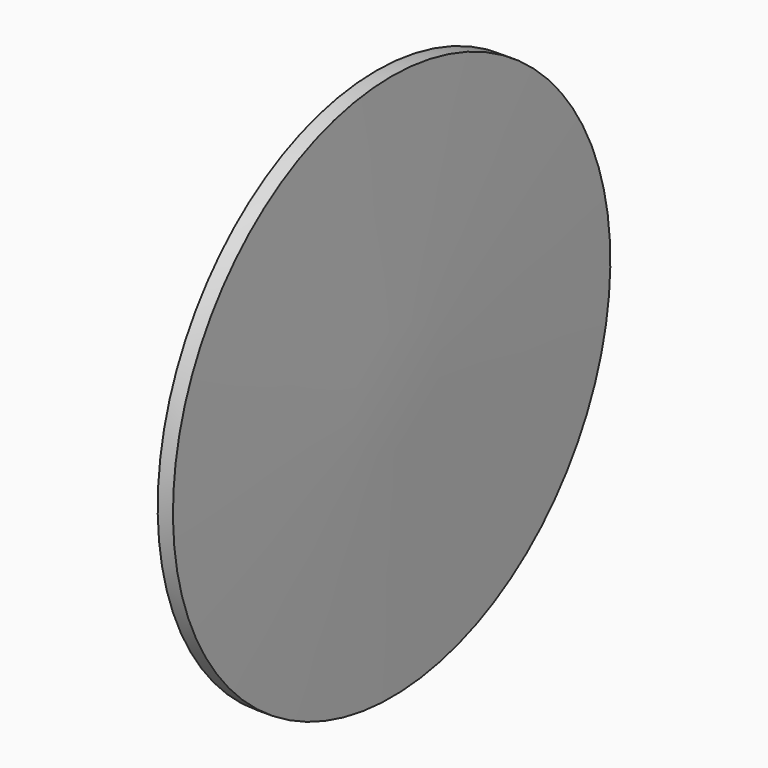
from build123d import *


# Not quite as in the source:
# - a feature names something its author has since deleted; it is built from what else it names


with BuildPart() as f1:
    # F0 (on Front) → F1 (revolve)
    with BuildSketch(Plane.XZ):
        Polygon((222.3129196464, 598.4423458588), (188.9083323345, 598.4423458588), (188.9083323345, 0), (234.95, 0), align=None)
    revolve(axis=Axis((0, 0, 0), (1, 0, 0)))


solid = f1.part
